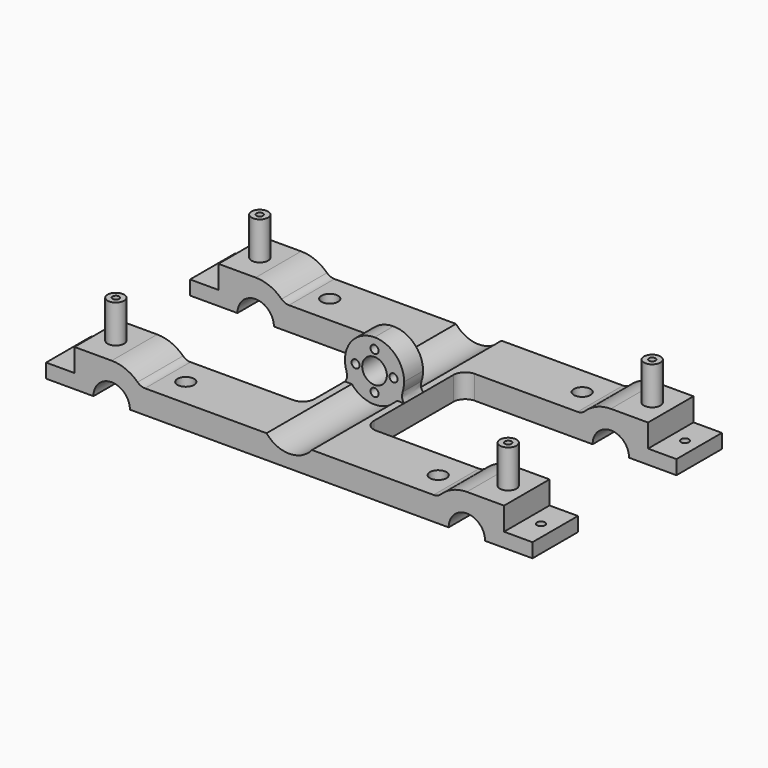
from build123d import *

# Parameters (mm, degrees)
F0_R      = 3.5
F1_DEPTH  = 10
F0_W      = 31.4
F0_H      = 24
F2_DEPTH  = 15.7
F3_DEPTH  = 30.5
F6_DEPTH  = 100
F7_R      = 1.7
F7_R_2    = 5.2
F8_DEPTH  = 60
F9_DEPTH  = 100
F10_DEPTH = 100
F11_DEPTH = 10
F12_R     = 5
F0_R_2    = 1.7
F13_DEPTH = 6
F14_DEPTH = 6
F15_R     = 3.5
F15_R_2   = 1.4
F16_DEPTH = 16


# Not quite as in the source:
# - a feature names something its author has since deleted; it is built from what else it names


with BuildPart() as f1:
    # F0 (on Top) → F1 (new body)
    with BuildSketch(Plane.XY):
        Polygon((59.3, 50), (0, 50), (-59.3, 50), (-59.3, 26), (-12.5, 26), (-12.5, 5), (12.5, 5), (12.5, 26), (59.3, 26), align=None)
        with Locations((-53.3, 38)):
            Circle(F0_R, mode=Mode.SUBTRACT)
        with Locations((53.3, 38)):
            Circle(F0_R, mode=Mode.SUBTRACT)
    extrude(amount=F1_DEPTH)

    # F0 (on Top) → F2 (join)
    with BuildSketch(Plane.XY):
        with Locations((-75, 38)):
            Rectangle(F0_W, F0_H)
        with Locations((75, 38)):
            Rectangle(F0_W, F0_H)
    extrude(amount=F2_DEPTH)



with BuildPart() as f1b:
    # F0 (on Top) → F1, piece 2 (new body)
    with BuildSketch(Plane.XY):
        Polygon((12.5, -5), (-12.5, -5), (-12.5, -26), (-59.3, -26), (-59.3, -50), (0, -50), (59.3, -50), (59.3, -26), (12.5, -26), align=None)
        with Locations((-53.3, -38)):
            Circle(F0_R, mode=Mode.SUBTRACT)
        with Locations((53.3, -38)):
            Circle(F0_R, mode=Mode.SUBTRACT)
    extrude(amount=F1_DEPTH)

    # F0 (on Top) → F2, piece 2 (join)
    with BuildSketch(Plane.XY):
        with Locations((-75, -38)):
            Rectangle(F0_W, F0_H)
        with Locations((75, -38)):
            Rectangle(F0_W, F0_H)
    extrude(amount=F2_DEPTH)


with BuildPart() as f1_1:
    add(f1.part)

    add(f1b.part)  # F3 merges F1b
    # F0 (on Top) → F3 (join)
    with BuildSketch(Plane.XY):
        Polygon((12.5, 5), (-12.5, 5), (-12.5, 0), (-12.5, -5), (12.5, -5), (12.5, 0), align=None)
    extrude(amount=F3_DEPTH)

    # F4: union 

    # F5 (on face) → F6 (cut)
    with BuildSketch(Plane.XZ.offset(50)):
        with BuildLine():
            Line((59.3, 15.7), (59.3, 10))
            Line((59.3, 10), (60.936808709, 10))
            ThreePointArc((60.936808709, 10), (62.6266035374, 10.3294327596), (64.0689074703, 11.2694816254))
            ThreePointArc((64.0689074703, 11.2694816254), (69.1025794418, 14.5502725321), (75, 15.7))
            Line((75, 15.7), (59.3, 15.7))
        make_face()
        with BuildLine():
            ThreePointArc((82.7, 0), (75, 7.7), (67.3, 0))
            Line((67.3, 0), (82.7, 0))
        make_face()
        with BuildLine():
            ThreePointArc((-75, 15.7), (-69.1025794418, 14.5502725321), (-64.0689074703, 11.2694816254))
            ThreePointArc((-64.0689074703, 11.2694816254), (-62.6266035374, 10.3294327596), (-60.936808709, 10))
            Line((-60.936808709, 10), (-59.3, 10))
            Line((-59.3, 10), (-59.3, 15.7))
            Line((-59.3, 15.7), (-75, 15.7))
        make_face()
        with BuildLine():
            ThreePointArc((-67.3, 0), (-75, 7.7), (-82.7, 0))
            Line((-82.7, 0), (-67.3, 0))
        make_face()
    extrude(amount=-F6_DEPTH, mode=Mode.SUBTRACT)

    # F7 (on face) → F8 (cut, symmetric)
    with BuildSketch(Plane.XZ.offset(5)):
        with BuildLine():
            Line((-12.5, 30.5), (-12.5, 18))
            ThreePointArc((-12.5, 18), (-8.8388347819, 26.8388347478), (-4.83e-08, 30.5))
            Line((-4.83e-08, 30.5), (-12.5, 30.5))
        make_face()
        with BuildLine():
            Line((12.5, 30.5), (-4.83e-08, 30.5))
            ThreePointArc((-4.83e-08, 30.5), (8.8388347478, 26.8388347819), (12.5, 18))
            Line((12.5, 18), (12.5, 30.5))
        make_face()
        with BuildLine():
            add(Edge.make_bspline(
                [(-11.8176156762, 13.9264315731), (-11.6747882381, 13.1368398711), (-11.3919431578, 11.6323543495), (-12.1435697242, 10.5264146596), (-12.5, 10)],
                knots=[0, 0, 0, 0, 0.5238869887, 1, 1, 1, 1], degree=3))
            ThreePointArc((-11.8176156762, 13.9264315731), (-12.3282236343, 15.9348360783), (-12.5, 18))
            Line((-12.5, 18), (-12.5, 10))
        make_face()
        with BuildLine():
            Line((12.5, 10), (12.5, 18))
            ThreePointArc((12.5, 18), (12.3282236343, 15.9348360783), (11.8176156762, 13.9264315731))
            add(Edge.make_bspline(
                [(11.8176156762, 13.9264315731), (11.6747882381, 13.1368398711), (11.3919431578, 11.6323543495), (12.1435697242, 10.5264146596), (12.5, 10)],
                knots=[0, 0, 0, 0, 0.5238869887, 1, 1, 1, 1], degree=3))
        make_face()
        with Locations((-8, 18)):
            Circle(F7_R)
        with Locations((0, 26)):
            Circle(F7_R)
        with Locations((8, 18)):
            Circle(F7_R)
        with BuildLine():
            ThreePointArc((1.7, 10), (0, 11.7), (-1.7, 10))
            Line((-1.7, 10), (1.7, 10))
        make_face()
        with BuildLine():
            Line((1.7, 10), (-1.7, 10))
            ThreePointArc((-1.7, 10), (0, 8.3), (1.7, 10))
        make_face()
        with Locations((0, 18)):
            Circle(F7_R_2)
    extrude(amount=F8_DEPTH, both=True, mode=Mode.SUBTRACT)

    # F7 (on face) → F9 (cut)
    with BuildSketch(Plane.XZ.offset(5)):
        with BuildLine():
            Line((-1.7, 10), (-9.6046863561, 10))
            ThreePointArc((-9.6046863561, 10), (0, 5.5), (9.6046863561, 10))
            Line((9.6046863561, 10), (1.7, 10))
            ThreePointArc((1.7, 10), (0, 8.3), (-1.7, 10))
        make_face()
    extrude(amount=F9_DEPTH, mode=Mode.SUBTRACT)

    # F7 (on face) → F10 (cut)
    with BuildSketch(Plane.XZ.offset(5)):
        with BuildLine():
            Line((-1.7, 10), (-9.6046863561, 10))
            ThreePointArc((-9.6046863561, 10), (0, 5.5), (9.6046863561, 10))
            Line((9.6046863561, 10), (1.7, 10))
            ThreePointArc((1.7, 10), (0, 8.3), (-1.7, 10))
        make_face()
    extrude(amount=-F10_DEPTH, mode=Mode.SUBTRACT)

    # F7 (on face) → F11 (join)
    with BuildSketch(Plane.XZ.offset(5)):
        with BuildLine():
            Line((-1.7, 10), (-9.6046863561, 10))
            ThreePointArc((-9.6046863561, 10), (0, 5.5), (9.6046863561, 10))
            Line((9.6046863561, 10), (1.7, 10))
            ThreePointArc((1.7, 10), (0, 8.3), (-1.7, 10))
        make_face()
    extrude(amount=-F11_DEPTH)

    # F12
    f12_edges = [f1_1.edges().sort_by_distance(p)[0] for p in [
        (-12.5, 26, 5),
        (12.5, 26, 5),
        (-12.5, -26, 5),
        (12.5, -26, 5),
    ]]
    fillet(f12_edges, radius=F12_R)

    # F0 (on Top) → F13 (join)
    with BuildSketch(Plane.XY):
        Polygon((-90.7, 26), (-90.7, 50), (-99.7, 50), (-102.7, 50), (-102.7, 26), (-99.7, 26), align=None)
        with Locations((-96.7, 38)):
            Circle(F0_R_2, mode=Mode.SUBTRACT)
        Polygon((-90.7, -50), (-90.7, -26), (-99.7, -26), (-102.7, -26), (-102.7, -50), (-99.7, -50), align=None)
        with Locations((-96.7, -38)):
            Circle(F0_R_2, mode=Mode.SUBTRACT)
        Polygon((99.7, -26), (90.7, -26), (90.7, -50), (99.7, -50), (102.7, -50), (102.7, -26), align=None)
        with Locations((96.7, -38)):
            Circle(F0_R_2, mode=Mode.SUBTRACT)
        Polygon((99.7, 50), (90.7, 50), (90.7, 26), (99.7, 26), (102.7, 26), (102.7, 50), align=None)
        with Locations((96.7, 38)):
            Circle(F0_R_2, mode=Mode.SUBTRACT)
    extrude(amount=F13_DEPTH)

    # F0 (on Top) → F14 (join)
    with BuildSketch(Plane.XY):
        with Locations((-53.3, 38)):
            Circle(F0_R)
        with Locations((-53.3, 38)):
            Circle(F0_R_2, mode=Mode.SUBTRACT)
        with Locations((53.3, 38)):
            Circle(F0_R)
        with Locations((53.3, 38)):
            Circle(F0_R_2, mode=Mode.SUBTRACT)
        with Locations((-53.3, -38)):
            Circle(F0_R)
        with Locations((-53.3, -38)):
            Circle(F0_R_2, mode=Mode.SUBTRACT)
        with Locations((53.3, -38)):
            Circle(F0_R)
        with Locations((53.3, -38)):
            Circle(F0_R_2, mode=Mode.SUBTRACT)
    extrude(amount=F14_DEPTH)

    # F15 (on face) → F16 (join)
    with BuildSketch(Plane.XY.offset(15.7)):
        with Locations((-82.85, 38)):
            Circle(F15_R)
        with Locations((-82.85, 38)):
            Circle(F15_R_2, mode=Mode.SUBTRACT)
        with Locations((82.85, 38)):
            Circle(F15_R)
        with Locations((82.85, 38)):
            Circle(F15_R_2, mode=Mode.SUBTRACT)
        with Locations((82.85, -38)):
            Circle(F15_R)
        with Locations((82.85, -38)):
            Circle(F15_R_2, mode=Mode.SUBTRACT)
        with Locations((-82.85, -38)):
            Circle(F15_R)
        with Locations((-82.85, -38)):
            Circle(F15_R_2, mode=Mode.SUBTRACT)
    extrude(amount=F16_DEPTH)


solid = f1_1.part
